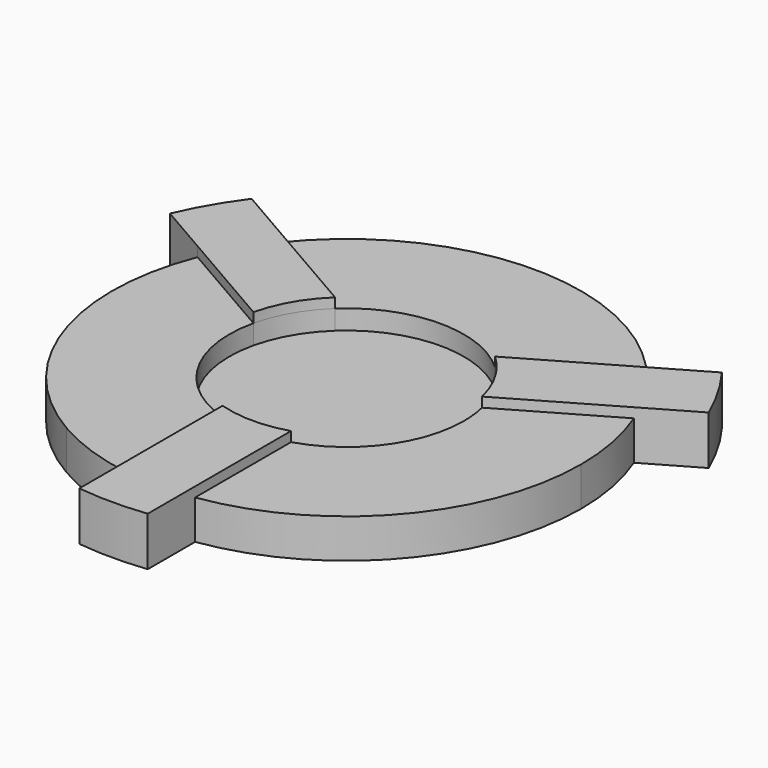
from build123d import *
from build123d import SkipClean  # not in build123d's __all__

# Parameters (mm, degrees)
F1_DEPTH = 25.4
F3_DEPTH = 12.7
F4_DEPTH = 6.35
F5_DEPTH = 31.75


# Not quite as in the source:
# - after a boolean that leaves OpenCascade's solid faulty, fix() repairs it


with BuildPart() as f1:
    # F0 (on Top) → F1 (new body)
    with BuildSketch(Plane.XY):
        with BuildLine():
            ThreePointArc((22.225, -150.7707178964), (115.3534784911, -99.5958583476), (152.4, 0))
            ThreePointArc((152.4, 0), (149.696971962, 28.5758041952), (141.6837718451, 56.1379443491))
            ThreePointArc((141.6837718451, 56.1379443491), (131.9822715367, 76.2), (119.4587718451, 94.6327735473))
            ThreePointArc((119.4587718451, 94.6327735473), (28.5758041952, 149.696971962), (-76.2, 131.9822715367))
            ThreePointArc((-76.2, 131.9822715367), (-99.5958583476, 115.3534784911), (-119.4587718451, 94.6327735473))
            ThreePointArc((-119.4587718451, 94.6327735473), (-131.9822715367, 76.2), (-141.6837718451, 56.1379443491))
            ThreePointArc((-141.6837718451, 56.1379443491), (-143.9292826863, -50.1011136144), (-76.2, -131.9822715367))
            ThreePointArc((-76.2, -131.9822715367), (-50.1011136144, -143.9292826863), (-22.225, -150.7707178964))
            ThreePointArc((-22.225, -150.7707178964), (0, -152.4), (22.225, -150.7707178964))
        make_face()
    extrude(amount=F1_DEPTH)

    # F2 (on face) → F3 (cut)
    with BuildSketch(Plane.XY.offset(25.4)):
        with BuildLine():
            ThreePointArc((22.225, -72.8868257986), (61.2371823323, -45.3480705212), (76.2, 0))
            ThreePointArc((76.2, 0), (75.7069908166, 8.6539899179), (74.2343427428, 17.1959983002))
            ThreePointArc((74.2343427428, 17.1959983002), (65.9911357684, 38.1), (52.0093427428, 55.6908274984))
            ThreePointArc((52.0093427428, 55.6908274984), (0, 76.2), (-52.0093427428, 55.6908274984))
            ThreePointArc((-52.0093427428, 55.6908274984), (-65.9911357684, 38.1), (-74.2343427428, 17.1959983002))
            ThreePointArc((-74.2343427428, 17.1959983002), (-65.9911357684, -38.1), (-22.225, -72.8868257986))
            ThreePointArc((-22.225, -72.8868257986), (0, -76.2), (22.225, -72.8868257986))
        make_face()
    extrude(amount=-F3_DEPTH, mode=Mode.SUBTRACT)

    # F2 (on face) → F4 (join)
    with BuildSketch(Plane.XY.offset(25.4)):
        with BuildLine():
            ThreePointArc((-74.2343427428, 17.1959983002), (-65.9911357684, 38.1), (-52.0093427428, 55.6908274984))
            Line((-52.0093427428, 55.6908274984), (-119.4587718451, 94.6327735473))
            ThreePointArc((-119.4587718451, 94.6327735473), (-131.9822715367, 76.2), (-141.6837718451, 56.1379443491))
            Line((-141.6837718451, 56.1379443491), (-74.2343427428, 17.1959983002))
        make_face()
        with BuildLine():
            Line((22.225, -150.7707178964), (22.225, -72.8868257986))
            ThreePointArc((22.225, -72.8868257986), (0, -76.2), (-22.225, -72.8868257986))
            Line((-22.225, -72.8868257986), (-22.225, -150.7707178964))
            ThreePointArc((-22.225, -150.7707178964), (0, -152.4), (22.225, -150.7707178964))
        make_face()
        with BuildLine():
            ThreePointArc((52.0093427428, 55.6908274984), (65.9911357684, 38.1), (74.2343427428, 17.1959983002))
            Line((74.2343427428, 17.1959983002), (141.6837718451, 56.1379443491))
            ThreePointArc((141.6837718451, 56.1379443491), (131.9822715367, 76.2), (119.4587718451, 94.6327735473))
            Line((119.4587718451, 94.6327735473), (52.0093427428, 55.6908274984))
        make_face()
    with SkipClean():  # cleaning this boolean's faces spoils the solid; the shape is the same uncleaned
        extrude(amount=F4_DEPTH)

    # F0 (on Top) → F5 (join)
    with BuildSketch(Plane.XY):
        with BuildLine():
            ThreePointArc((119.4587718451, 94.6327735473), (131.9822715367, 76.2), (141.6837718451, 56.1379443491))
            Line((141.6837718451, 56.1379443491), (174.9637268225, 75.3521353139))
            ThreePointArc((174.9637268225, 75.3521353139), (164.9778394209, 95.25), (152.7387268225, 113.8469645122))
            Line((152.7387268225, 113.8469645122), (119.4587718451, 94.6327735473))
        make_face()
        with BuildLine():
            ThreePointArc((-141.6837718451, 56.1379443491), (-131.9822715367, 76.2), (-119.4587718451, 94.6327735473))
            Line((-119.4587718451, 94.6327735473), (-152.7387268225, 113.8469645122))
            ThreePointArc((-152.7387268225, 113.8469645122), (-164.9778394209, 95.25), (-174.9637268225, 75.3521353139))
            Line((-174.9637268225, 75.3521353139), (-141.6837718451, 56.1379443491))
        make_face()
        with BuildLine():
            Line((22.225, -189.1990998261), (22.225, -150.7707178964))
            ThreePointArc((22.225, -150.7707178964), (0, -152.4), (-22.225, -150.7707178964))
            Line((-22.225, -150.7707178964), (-22.225, -189.1990998261))
            ThreePointArc((-22.225, -189.1990998261), (0, -190.5), (22.225, -189.1990998261))
        make_face()
    extrude(amount=F5_DEPTH)

    add(f1.part.fix(), mode=Mode.REPLACE)


solid = f1.part
